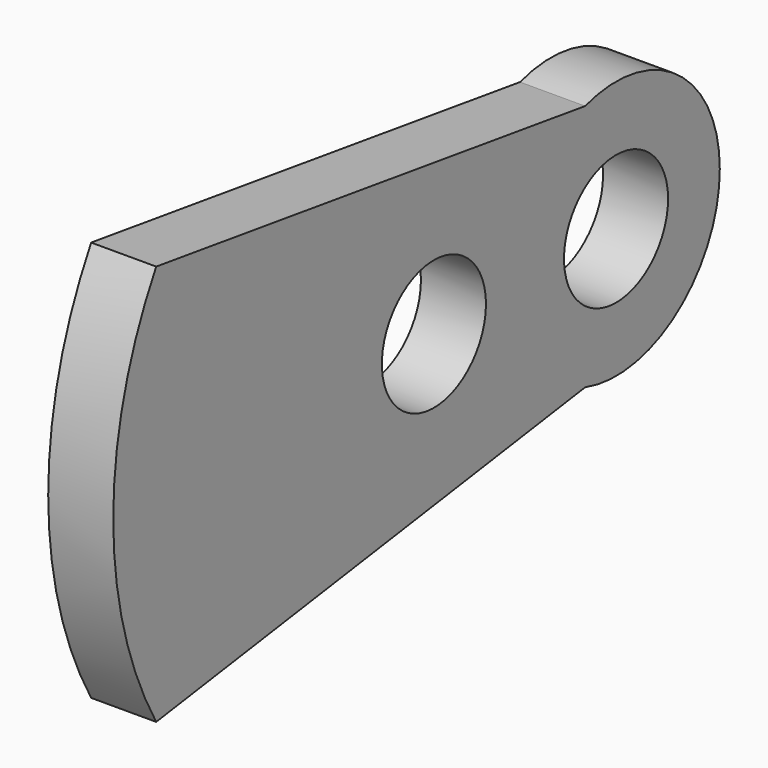
from build123d import *

# Parameters (mm, degrees)
F0_R     = 12.7
F1_DEPTH = 12.7


# Not quite as in the source:
# - a length typed as a fraction of an inch, garbled in the dataset ("3 / 203.2 mm" for 3/8 in), is restored


with BuildPart() as f1:
    # F0 (on Right) → F1 (new body)
    with BuildSketch(Plane.YZ):
        with BuildLine():
            ThreePointArc((36.9027980984, -24.1696875), (19.129375, 0), (36.9027980984, 24.1696875))
            Line((36.9027980984, 24.1696875), (-67.7783956954, 39.131875))
            ThreePointArc((-67.7783956954, 39.131875), (-78.26375, 0), (-67.7783956954, -39.131875))
            Line((-67.7783956954, -39.131875), (36.9027980984, -24.1696875))
        make_face()
        Circle(F0_R, mode=Mode.SUBTRACT)
        with BuildLine():
            ThreePointArc((36.9027980984, -24.1696875), (59.4505696765, -20.3989450651), (69.770625, 0))
            ThreePointArc((69.770625, 0), (59.4505696765, 20.3989450651), (36.9027980984, 24.1696875))
            ThreePointArc((36.9027980984, 24.1696875), (19.129375, 0), (36.9027980984, -24.1696875))
        make_face()
        with Locations((44.45, 0)):
            Circle(F0_R, mode=Mode.SUBTRACT)
    extrude(amount=F1_DEPTH)


solid = f1.part
